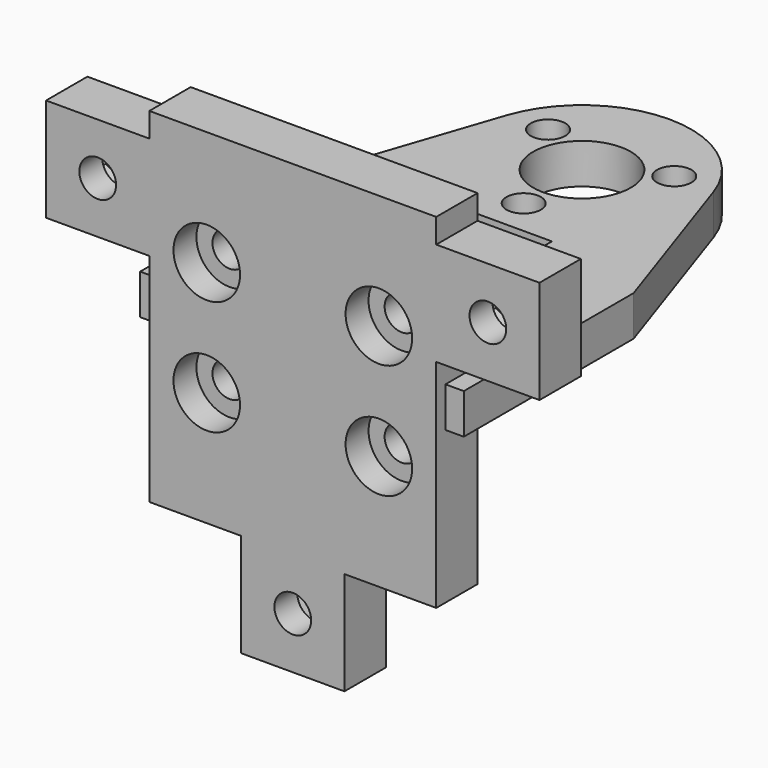
from build123d import *

# Parameters (mm, degrees)
F0_R          = 1.5
F0_R_2        = 4.25
F1_DEPTH      = 3.5
F2_R          = 1.5
F2_W          = 9
F2_H          = 9
F2_R_2        = 1.6
F2_W_2        = 25
F2_H_2        = 3.5
F3_DEPTH      = 3.5
F3_DEPTH_BACK = 1
F4_R          = 1.6
F5_DEPTH      = 2
F6_R          = 2.9
F6_R_2        = 1.5
F7_DEPTH      = 2.5


# Not quite as in the source:
# - a feature names something its author has since deleted; it is built from what else it names


with BuildPart() as f1:
    # F0 (on Top) → F1 (new body)
    with BuildSketch(Plane.XY):
        with BuildLine():
            Line((-14.1, -30.5), (0, -30.5))
            Line((0, -30.5), (14.1, -30.5))
            Line((14.1, -30.5), (14.1, -12))
            Line((14.1, -12), (9.025382269, 3.044355416))
            ThreePointArc((9.025382269, 3.044355416), (0, 9.525), (-9.025382269, 3.044355416))
            Line((-9.025382269, 3.044355416), (-14.1, -12))
            Line((-14.1, -12), (-14.1, -30.5))
        make_face()
        Polygon((10.2, -27), (0, -27), (-10.2, -27), (-10.2, -18.95), (-5, -18.95), (-5, -9.525), (0, -9.525), (5, -9.525), (5, -18.95), (10.2, -18.95), align=None, mode=Mode.SUBTRACT)
        with Locations((-5.499261314, 3.175)):
            Circle(F0_R, mode=Mode.SUBTRACT)
        with Locations((0, -6.35)):
            Circle(F0_R, mode=Mode.SUBTRACT)
        Circle(F0_R_2, mode=Mode.SUBTRACT)
        with Locations((5.499261314, 3.175)):
            Circle(F0_R, mode=Mode.SUBTRACT)
    extrude(amount=F1_DEPTH)

    # F2 (on face) → F3 (join, two sides)
    with BuildSketch(Plane.XZ.offset(30.5)) as f3_sk:
        Polygon((12.5, 16.75), (-12.5, 16.75), (-12.5, 14.625), (-12.5, 5.625), (-12.5, 3.5), (12.5, 3.5), (12.5, 5.625), (12.5, 14.625), align=None)
        with Locations((-7.5, 6.75)):
            Circle(F2_R, mode=Mode.SUBTRACT)
        with Locations((7.5, 6.75)):
            Circle(F2_R, mode=Mode.SUBTRACT)
        Polygon((12.5, 0), (-12.5, 0), (-12.5, -13.25), (-4.5, -13.25), (4.5, -13.25), (12.5, -13.25), align=None)
        with Locations((-7.5, -3.25)):
            Circle(F2_R, mode=Mode.SUBTRACT)
        with Locations((7.5, -3.25)):
            Circle(F2_R, mode=Mode.SUBTRACT)
        with Locations((-17, 10.125)):
            Rectangle(F2_W, F2_H)
        with Locations((-17, 10.125)):
            Circle(F2_R_2, mode=Mode.SUBTRACT)
        with Locations((17, 10.125)):
            Rectangle(F2_W, F2_H)
        with Locations((17, 10.125)):
            Circle(F2_R_2, mode=Mode.SUBTRACT)
        with Locations((0, -17.75)):
            Rectangle(F2_W, F2_H)
        with Locations((0, -17.75)):
            Circle(F2_R_2, mode=Mode.SUBTRACT)
        with Locations((0, 1.75)):
            Rectangle(F2_W_2, F2_H_2)
    extrude(amount=-F3_DEPTH)
    extrude(f3_sk.sketch, amount=F3_DEPTH_BACK)

    # F4 (on face) → F5 (cut)
    with BuildSketch(Plane(origin=(0, -27, 0), x_dir=(-1, 0, 0), z_dir=(0, 1, 0))):
        Polygon((-19.9, 11.7993157806), (-19.9, 8.4506842194), (-17, 6.7763684387), (-14.1, 8.4506842194), (-14.1, 11.7993157806), (-17, 13.4736315613), align=None)
        with Locations((-17, 10.125)):
            Circle(F4_R, mode=Mode.SUBTRACT)
        Polygon((17, 13.4736315613), (14.1, 11.7993157806), (14.1, 8.4506842194), (17, 6.7763684387), (19.9, 8.4506842194), (19.9, 11.7993157806), align=None)
        with Locations((17, 10.125)):
            Circle(F4_R, mode=Mode.SUBTRACT)
        Polygon((1.6743157806, -14.85), (-1.6743157806, -14.85), (-3.3486315613, -17.75), (-1.6743157806, -20.65), (1.6743157806, -20.65), (3.3486315613, -17.75), align=None)
        with Locations((0, -17.75)):
            Circle(F4_R, mode=Mode.SUBTRACT)
    extrude(amount=-F5_DEPTH, mode=Mode.SUBTRACT)

    # F6 (on face) → F7 (cut)
    with BuildSketch(Plane.XZ.offset(31.5)):
        with Locations((-7.5, 6.75)):
            Circle(F6_R)
        with Locations((-7.5, 6.75)):
            Circle(F6_R_2, mode=Mode.SUBTRACT)
        with Locations((7.5, 6.75)):
            Circle(F6_R)
        with Locations((7.5, 6.75)):
            Circle(F6_R_2, mode=Mode.SUBTRACT)
        with Locations((7.5, -3.25)):
            Circle(F6_R)
        with Locations((7.5, -3.25)):
            Circle(F6_R_2, mode=Mode.SUBTRACT)
        with Locations((-7.5, -3.25)):
            Circle(F6_R)
        with Locations((-7.5, -3.25)):
            Circle(F6_R_2, mode=Mode.SUBTRACT)
    extrude(amount=-F7_DEPTH, mode=Mode.SUBTRACT)


solid = f1.part
